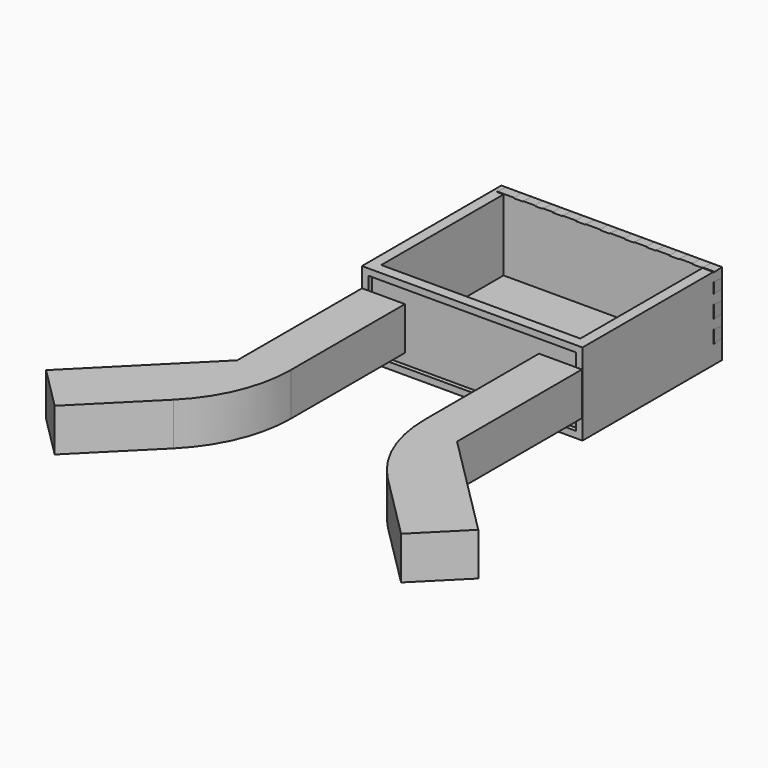
from build123d import *

# Parameters (mm, degrees)
F0_W         = 50.8
F0_H         = 50.8
F1_DEPTH     = 235.585
F2_SIZE      = 50.79999
F3_SIZE      = 50.79999
F4_W         = 71.8420489686
F4_H         = 50.8
F6_DEPTH     = 177.8
F5_W         = 71.8420489686
F5_H         = 50.8
F7_DEPTH     = 177.8
F8_R         = 161.8478442459
F8_2_R       = 161.8478442459
F9_W         = 261.1634731293
F9_H         = 97.1325188875
F10_DEPTH    = 206.375
F11_T        = -12.7
F12_T        = 7.62
F12_T3_DEPTH = 99.6725188875
F12_T5_DEPTH = 196.215
F12_T7_DEPTH = 251.0034731293
F14_DEPTH    = 12.7
F14_TAPER    = -3


# Not quite as in the source:
# - a fillet or chamfer is up to 0.001 mm smaller than in the source, because OpenCascade refuses the exact size
# - a shell that OpenCascade refuses in one call is made with other operations: the cavity is built on its own and cut out


with BuildPart() as f1:
    # F0 (on Front) → F1 (new body)
    with BuildSketch(Plane.XZ):
        with Locations((-105.0636373861, 0)):
            Rectangle(F0_W, F0_H)
    extrude(amount=F1_DEPTH)

    # F3 (size 50.8 in the source; OpenCascade refuses exactly that, so slightly less here)
    f3_edges = [f1.edges().sort_by_distance(p)[0] for p in [
        (-130.463637, -235.585, 0),
    ]]
    chamfer(f3_edges, length=F3_SIZE)

    # F4 (on face) → F6 (join)
    with BuildSketch(Plane(origin=(-157.624318693, -157.624318693, 0), x_dir=(0.7071067812, -0.7071067812, 0), z_dir=(-0.7071067812, -0.7071067812, 0))):
        with Locations((74.3320283519, 0)):
            Rectangle(F4_W, F4_H)
    extrude(amount=F6_DEPTH)

    # F8
    f8_edges = [f1.edges().sort_by_distance(p)[0] for p in [
        (-79.663647, -235.585, 0),
    ]]
    fillet(f8_edges, radius=F8_R)


with BuildPart() as f1b:
    # F0 (on Front) → F1, piece 2 (new body)
    with BuildSketch(Plane.XZ):
        with Locations((104.4863691024, 0)):
            Rectangle(F0_W, F0_H)
    extrude(amount=F1_DEPTH)

    # F2 (size 50.8 in the source; OpenCascade refuses exactly that, so slightly less here)
    f2_edges = [f1b.edges().sort_by_distance(p)[0] for p in [
        (129.886369, -235.585, 0),
    ]]
    chamfer(f2_edges, length=F2_SIZE)

    # F5 (on face) → F7 (join)
    with BuildSketch(Plane(origin=(157.3356845512, -157.3356845512, 0), x_dir=(0.7071067812, 0.7071067812, 0), z_dir=(0.7071067812, -0.7071067812, 0))):
        with Locations((-74.7402186698, 0)):
            Rectangle(F5_W, F5_H)
    extrude(amount=F7_DEPTH)

    # F8#2
    f8_2_edges = [f1b.edges().sort_by_distance(p)[0] for p in [
        (79.086379, -235.585, 0),
    ]]
    fillet(f8_2_edges, radius=F8_2_R)


with BuildPart() as f10:
    # F9 (on Front) → F10 (new body)
    with BuildSketch(Plane.XZ):
        Rectangle(F9_W, F9_H)
    extrude(amount=-F10_DEPTH)

    # F11
    f11_openings = [f10.faces().sort_by_distance(p)[0] for p in [
        (0, 103.1875, 48.566259),
    ]]
    offset(amount=F11_T, openings=f11_openings)

    # F12: shell of thickness 7.62, made by hand


with BuildPart() as f12_core1:
    # F12_t2: copy of F10
    add(f10.part)

    # the walls: a layer under each face that stays
    f12_faces = [f12_core1.faces().sort_by_distance(p)[0] for p in [
        (-130.5817365646, 103.1875, 0),
        (0, 103.1875, -48.5662594438),
        (130.5817365646, 103.1875, 0),
        (0, 206.375, 0),
        (121.8762874603, 199.4958333333, 48.5662594438),
        (117.8817365646, 103.1875, 6.35),
        (-117.8817365646, 103.1875, 6.35),
        (0, 12.7, 6.35),
        (0, 193.675, 6.35),
        (0, 103.1875, -35.8662594438),
    ]]
    thicken(f12_faces, amount=-F12_T, mode=Mode.SUBTRACT)

    # F12_s4 → F12_t3 (cut)
    with BuildSketch(Plane.XY.offset(-43.4862594438)):
        Polygon((117.8055365646, 12.7762), (125.5017365646, 12.7), (125.5017365646, 5.08), (117.8817365646, 5.08), align=None)
        Polygon((117.8055365646, 193.5988), (125.5017365646, 193.675), (125.5017365646, 201.295), (117.8817365646, 201.295), align=None)
        Polygon((-117.8055365646, 193.5988), (-125.5017365646, 193.675), (-125.5017365646, 201.295), (-117.8817365646, 201.295), align=None)
        Polygon((-117.8055365646, 12.7762), (-125.5017365646, 12.7), (-125.5017365646, 5.08), (-117.8817365646, 5.08), align=None)
    extrude(amount=F12_T3_DEPTH, mode=Mode.SUBTRACT)

    # F12_s6 → F12_t5 (cut)
    with BuildSketch(Plane.XZ.offset(-201.295)):
        Polygon((117.8055365646, -35.7900594438), (125.5017365646, -35.8662594438), (125.5017365646, -43.4862594438), (117.8817365646, -43.4862594438), align=None)
        Polygon((-117.8055365646, -35.7900594438), (-125.5017365646, -35.8662594438), (-125.5017365646, -43.4862594438), (-117.8817365646, -43.4862594438), align=None)
    extrude(amount=F12_T5_DEPTH, mode=Mode.SUBTRACT)

    # F12_s8 → F12_t7 (cut)
    with BuildSketch(Plane.YZ.offset(-125.5017365646)):
        Polygon((12.7762, -35.7900594438), (5.08, -35.8662594438), (5.08, -43.4862594438), (12.7, -43.4862594438), align=None)
        Polygon((193.5988, -35.7900594438), (201.295, -35.8662594438), (201.295, -43.4862594438), (193.675, -43.4862594438), align=None)
    extrude(amount=F12_T7_DEPTH, mode=Mode.SUBTRACT)


with BuildPart() as f10_1:
    add(f10.part)

    # what is left inside the walls is the cavity
    f12_cavity = [f12_core1.part.solids().sort_by_distance(p)[0] for p in [
        (0, 5.0038, 13.648753),
    ]]
    add(f12_cavity, mode=Mode.SUBTRACT)

    # F13 (on face) → F14 (join)
    with BuildSketch(Plane(origin=(0, 206.375, 0), x_dir=(-1, 0, 0), z_dir=(0, 1, 0))):
        Polygon((-130.5817365646, -12.7628296614), (-130.5817365646, -25.839349255), (-107.140854001, -48.5662594438), (-92.2972410917, -48.5662594438), align=None)
        Polygon((-130.5817365646, 13.3902104571), (-130.5817365646, 0), (-77.1002024412, -48.5662594438), (-62.9634261131, -48.5662594438), align=None)
        Polygon((-130.5817365646, 37.0693132281), (-130.5817365646, 26.1133126915), (-48.826649785, -48.5662594438), (-36.1035428941, -48.5662594438), align=None)
        Polygon((-118.096858263, 48.5662594438), (-130.5817365646, 48.5662594438), (-21.6133445501, -48.5662594438), (-9.2436661944, -48.5662594438), align=None)
        Polygon((-90.5301421881, 48.5662594438), (-104.6669185162, 48.5662594438), (4.8931078054, -48.5662594438), (17.2627996653, -48.5662594438), align=None)
        Polygon((-62.9634261131, 48.5662594438), (-77.8070390224, 48.5662594438), (32.4598327279, -48.5662594438), (45.1829358935, -48.5662594438), align=None)
        Polygon((-37.1638014913, 48.5662594438), (-50.2403229475, 48.5662594438), (58.9662902057, -48.5662594438), (72.3962336779, -48.5662594438), align=None)
        Polygon((-8.5065541789, 48.5662594438), (-24.087285623, 48.5662594438), (89.0069380403, -48.5662594438), (101.9576340914, -48.5662594438), align=None)
        Polygon((20.2443990856, 48.5662594438), (4.6079140157, 48.5662594438), (116.3331121206, -48.5662594438), (130.5817365646, -48.5662594438), align=None)
        Polygon((47.7343462408, 48.5662594438), (33.3588682115, 48.5662594438), (130.5817365646, -38.4523272514), (130.5817365646, -24.8334556818), align=None)
        Polygon((70.9368661046, 48.5662594438), (60.5966113508, 48.5662594438), (130.5817365646, -13.9887984842), (130.5817365646, -5.4139527492), align=None)
        Polygon((94.3915918469, 48.5662594438), (82.0337310433, 48.5662594438), (130.5817365646, 4.6741003171), (130.5817365646, 17.2841660678), align=None)
        Polygon((124.9079555273, 48.5662594438), (107.0016622543, 48.5662594438), (130.5817365646, 31.1552416533), (130.5817365646, 43.7653101981), align=None)
    extrude(amount=-F14_DEPTH, taper=F14_TAPER)


solid = Compound([f1.part, f1b.part, f10_1.part])
